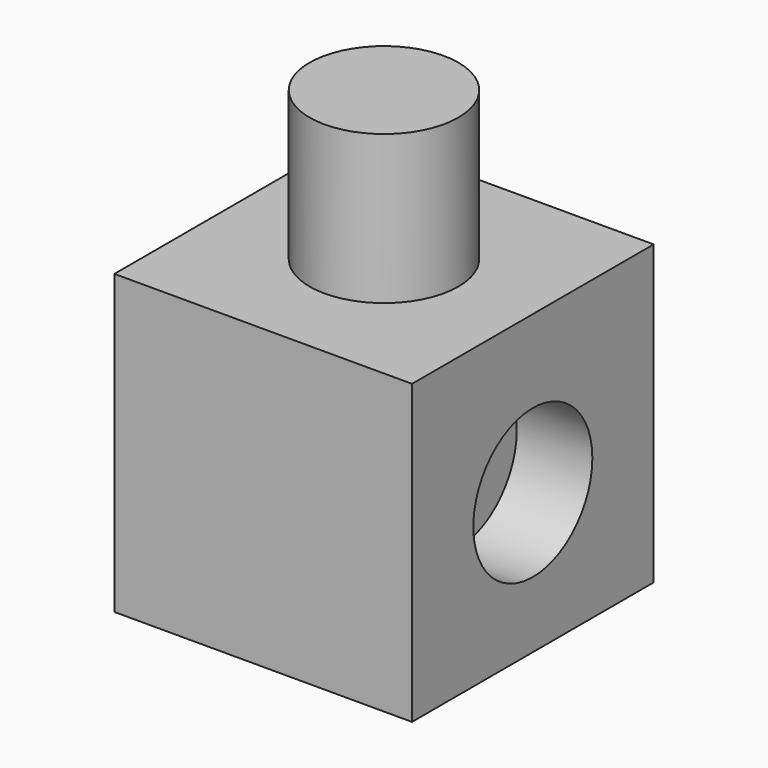
from build123d import *

# Parameters (mm, degrees)
F0_W     = 100
F0_H     = 101.4652305061
F1_DEPTH = 100
F2_R     = 25
F3_DEPTH = 50
F4_R     = 25
F5_DEPTH = 50
F7_DEPTH = 25.4
F8_R     = 25
F9_DEPTH = 25.4


# Not quite as in the source:
# - the program builds the solid bodies; features that only make, move or delete a surface that nothing else refers to are left out


with BuildPart() as f1:
    # F0 (on Top) → F1 (new body)
    with BuildSketch(Plane.XY):
        Rectangle(F0_W, F0_H)
    extrude(amount=F1_DEPTH)

    # F2 (on face) → F3 (join)
    with BuildSketch(Plane.XY.offset(100)):
        Circle(F2_R)
    extrude(amount=F3_DEPTH)

    # F4 (on Top) → F5 (join)
    with BuildSketch(Plane.XY):
        Circle(F4_R)
    extrude(amount=F5_DEPTH)

    # F4 (on Top) → F7 (join)
    with BuildSketch(Plane.XY):
        Circle(F4_R)
    extrude(amount=F7_DEPTH)

    # F8 (on face) → F9 (cut)
    with BuildSketch(Plane.YZ.offset(50)):
        with Locations((0, 47.2276035258)):
            Circle(F8_R)
    extrude(amount=-F9_DEPTH, mode=Mode.SUBTRACT)


solid = f1.part
